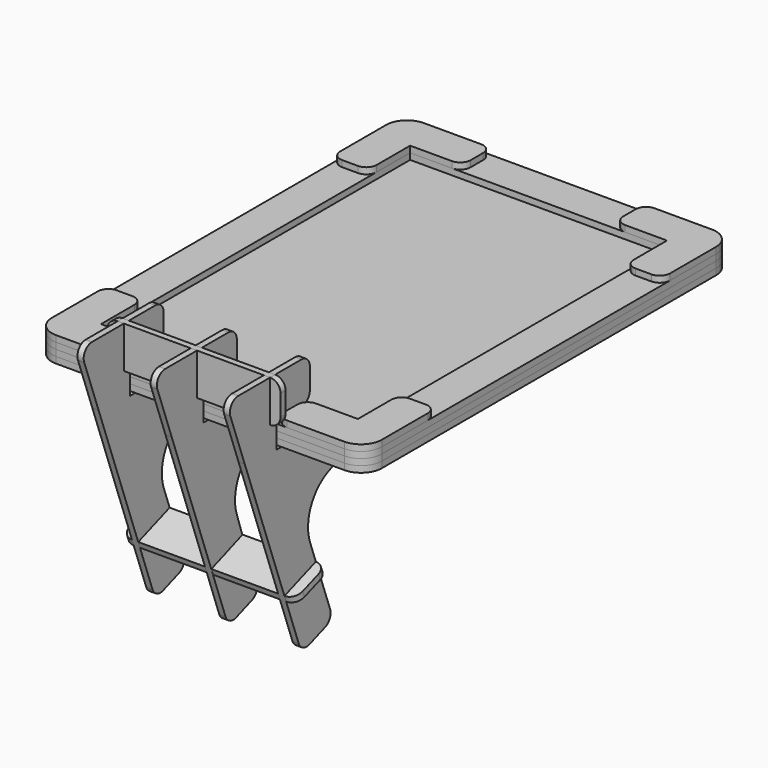
from build123d import *

# Parameters (mm, degrees)
F1_DEPTH  = 3
F3_R      = 6
F3_W      = 123
F3_H      = 185
F4_DEPTH  = 3
F5_R      = 6
F5_W      = 123
F5_H      = 185
F6_DEPTH  = 3
F9_DEPTH  = 1.5
F11_DEPTH = 1.5
F17_DEPTH = 3
F22_DEPTH = 3
F25_DEPTH = 3
F27_DEPTH = 3


# Not quite as in the source:
# - ends of sketch curves that miss each other by under 0.0002 mm in the source are joined


with BuildPart() as f1:
    # F0 (on Top) → F1 (new body)
    with BuildSketch(Plane.XY):
        with BuildLine():
            Line((-69, -110), (69, -110))
            ThreePointArc((69, -110), (76.0710678119, -107.0710678119), (79, -100))
            Line((79, -100), (79, 100))
            ThreePointArc((79, 100), (76.0710678119, 107.0710678119), (69, 110))
            Line((69, 110), (-69, 110))
            ThreePointArc((-69, 110), (-76.0710678119, 107.0710678119), (-79, 100))
            Line((-79, 100), (-79, -100))
            ThreePointArc((-79, -100), (-76.0710678119, -107.0710678119), (-69, -110))
        make_face()
    extrude(amount=F1_DEPTH)


with BuildPart() as f4:
    # F3 (on offset) → F4 (new body)
    with BuildSketch(Plane.XY.offset(3)):
        with BuildLine():
            Line((-69, -110), (69, -110))
            ThreePointArc((69, -110), (76.0710678119, -107.0710678119), (79, -100))
            Line((79, -100), (79, 100))
            ThreePointArc((79, 100), (76.0710678119, 107.0710678119), (69, 110))
            Line((69, 110), (-69, 110))
            ThreePointArc((-69, 110), (-76.0710678119, 107.0710678119), (-79, 100))
            Line((-79, 100), (-79, -100))
            ThreePointArc((-79, -100), (-76.0710678119, -107.0710678119), (-69, -110))
        make_face()
        with Locations((-68.7855339059, -99.7855339059)):
            Circle(F3_R, mode=Mode.SUBTRACT)
        with Locations((68.7855339059, -99.7855339059)):
            Circle(F3_R, mode=Mode.SUBTRACT)
        with Locations((-68.7855339059, 99.7855339059)):
            Circle(F3_R, mode=Mode.SUBTRACT)
        Rectangle(F3_W, F3_H, mode=Mode.SUBTRACT)
        with Locations((68.7855339059, 99.7855339059)):
            Circle(F3_R, mode=Mode.SUBTRACT)
    extrude(amount=F4_DEPTH)


with BuildPart() as f6:
    # F5 (on face) → F6 (new body)
    with BuildSketch(Plane(origin=(0, 0, 0), x_dir=(1, 0, 0), z_dir=(0, 0, -1))):
        with BuildLine():
            Line((-69, -110), (69, -110))
            ThreePointArc((69, -110), (76.0710678119, -107.0710678119), (79, -100))
            Line((79, -100), (79, 100))
            ThreePointArc((79, 100), (76.0710678119, 107.0710678119), (69, 110))
            Line((69, 110), (-69, 110))
            ThreePointArc((-69, 110), (-76.0710678119, 107.0710678119), (-79, 100))
            Line((-79, 100), (-79, -100))
            ThreePointArc((-79, -100), (-76.0710678119, -107.0710678119), (-69, -110))
        make_face()
        with Locations((-68.7855339059, -99.7855339059)):
            Circle(F5_R, mode=Mode.SUBTRACT)
        with Locations((68.7855339059, -99.7855339059)):
            Circle(F5_R, mode=Mode.SUBTRACT)
        with Locations((-68.7855339059, 99.7855339059)):
            Circle(F5_R, mode=Mode.SUBTRACT)
        Rectangle(F5_W, F5_H, mode=Mode.SUBTRACT)
        with Locations((68.7855339059, 99.7855339059)):
            Circle(F5_R, mode=Mode.SUBTRACT)
    extrude(amount=F6_DEPTH)


with BuildPart() as f9:
    # F8 (on offset) → F9 (new body, symmetric)
    with BuildSketch(Plane.YZ.offset(35)):
        with BuildLine():
            Line((-110, -5), (-110, 7))
            Line((-110, 7), (-95, 7))
            ThreePointArc((-95, 7), (-91.4644660941, 8.4644660941), (-90, 12))
            Line((-90, 12), (-90, 22))
            ThreePointArc((-90, 22), (-91.4644660941, 25.5355339059), (-95, 27))
            Line((-95, 27), (-111, 27))
            Line((-111, 27), (-111, 17))
            Line((-111, 17), (-113.8, 17))
            Line((-113.8, 17), (-113.8, 27))
            Line((-113.8, 27), (-132.8592599663, 27))
            ThreePointArc((-132.8592599663, 27), (-136.9550201877, 24.8678821818), (-137.5577230702, 20.2898992834))
            Line((-137.5577230702, 20.2898992834), (-128.9215966854, -3.4376629506))
            Line((-128.9215966854, -3.4376629506), (-96.6636040684, -92.0657692625))
            ThreePointArc((-96.6636040684, -92.0657692625), (-94.0782322732, -94.8872074811), (-90.2550402479, -95.0541316498))
            Line((-90.2550402479, -95.0541316498), (-80.85811404, -91.6339302166))
            ThreePointArc((-80.85811404, -91.6339302166), (-78.0366758215, -89.0485584213), (-77.8697516527, -85.225366396))
            Line((-77.8697516527, -85.225366396), (-85.4625988345, -64.3641902146))
            Line((-85.4625988345, -64.3641902146), (-94.8595250424, -67.7843916478))
            Line((-94.8595250424, -67.7843916478), (-95.8171814437, -65.1532523096))
            Line((-95.8171814437, -65.1532523096), (-86.4202552359, -61.7330508764))
            Line((-86.4202552359, -61.7330508764), (-89.8404566691, -52.3361246685))
            ThreePointArc((-89.8404566691, -52.3361246685), (-87.3851192861, -33.685985643), (-70.6994961108, -25))
            Line((-70.6994961108, -25), (-57.8, -24.9999998882))
            Line((-57.8, -24.9999998882), (-57.8, -14.9999998882))
            Line((-57.8, -14.9999998882), (-55, -14.9999998882))
            Line((-55, -14.9999998882), (-55, -24.9999998882))
            Line((-55, -24.9999998882), (-30, -24.9999998882))
            ThreePointArc((-30, -24.9999998882), (-26.4644660941, -23.5355337942), (-25, -19.9999998882))
            Line((-25, -19.9999998882), (-25, -6.9999998882))
            ThreePointArc((-25, -6.9999998882), (-26.4644660941, -3.4644659823), (-30, -1.9999998882))
            Line((-30, -1.9999998882), (-43.5, -1.9999998882))
            ThreePointArc((-43.5, -1.9999998882), (-44.5606601718, -2.4393397165), (-45, -3.4999998882))
            ThreePointArc((-45, -3.4999998882), (-45.4393398282, -4.56066006), (-46.5, -4.9999998882))
            Line((-46.5, -4.9999998882), (-110, -5))
        make_face()
    extrude(amount=F9_DEPTH, both=True)


with BuildPart() as f11:
    # F10 (on Right) → F11 (new body, symmetric)
    with BuildSketch(Plane.YZ):
        with BuildLine():
            Line((-110.7523969784, -8.8638670102), (-110.7523969784, 3.1361329898))
            Line((-110.7523969784, 3.1361329898), (-95.7523969784, 3.1361329898))
            ThreePointArc((-95.7523969784, 3.1361329898), (-92.2168630724, 4.6005990838), (-90.7523969784, 8.1361329898))
            Line((-90.7523969784, 8.1361329898), (-90.7523969784, 18.1361329898))
            ThreePointArc((-90.7523969784, 18.1361329898), (-92.2168630724, 21.6716668957), (-95.7523969784, 23.1361329898))
            Line((-95.7523969784, 23.1361329898), (-111.7523969784, 23.1361329898))
            Line((-111.7523969784, 23.1361329898), (-111.7523969784, 13.1361329898))
            Line((-111.7523969784, 13.1361329898), (-114.5523969784, 13.1361329898))
            Line((-114.5523969784, 13.1361329898), (-114.5523969784, 23.1361329898))
            Line((-114.5523969784, 23.1361329898), (-133.6116569447, 23.1361329898))
            ThreePointArc((-133.6116569447, 23.1361329898), (-137.7074171661, 21.0040151715), (-138.3101200486, 16.4260322731))
            Line((-138.3101200486, 16.4260322731), (-129.6739936637, -7.3015299608))
            Line((-129.6739936637, -7.3015299608), (-97.5212095615, -95.9682632155))
            ThreePointArc((-97.5212095615, -95.9682632155), (-94.9200677452, -98.7751693757), (-91.096000348, -98.9206667385))
            Line((-91.096000348, -98.9206667385), (-81.7183876115, -95.4478610478))
            ThreePointArc((-81.7183876115, -95.4478610478), (-78.9114814514, -92.8467192315), (-78.7659840886, -89.0226518343))
            Line((-78.7659840886, -89.0226518343), (-86.4756127218, -68.2043515593))
            Line((-86.4756127218, -68.2043515593), (-95.8532254583, -71.6771572499))
            Line((-95.8532254583, -71.6771572499), (-96.8256110516, -69.0514256837))
            Line((-96.8256110516, -69.0514256837), (-87.4479983152, -65.5786199931))
            Line((-87.4479983152, -65.5786199931), (-90.5928536475, -56.1999916787))
            ThreePointArc((-90.5928536475, -56.1999916787), (-88.1375162644, -37.5498526532), (-71.4518930892, -28.8638670102))
            Line((-71.4518930892, -28.8638670102), (-58.5523969784, -28.8638670102))
            Line((-58.5523969784, -28.8638670102), (-58.5523969784, -18.8638670102))
            Line((-58.5523969784, -18.8638670102), (-55.7523969784, -18.8638670102))
            Line((-55.7523969784, -18.8638670102), (-55.7523969784, -28.8638670102))
            Line((-55.7523969784, -28.8638670102), (-30.7523969784, -28.8638670102))
            ThreePointArc((-30.7523969784, -28.8638670102), (-27.2168630724, -27.3994009162), (-25.7523969784, -23.8638670102))
            Line((-25.7523969784, -23.8638670102), (-25.7523969784, -10.8638670102))
            ThreePointArc((-25.7523969784, -10.8638670102), (-27.2168630724, -7.3283331043), (-30.7523969784, -5.8638670102))
            Line((-30.7523969784, -5.8638670102), (-44.2523969784, -5.8638670102))
            ThreePointArc((-44.2523969784, -5.8638670102), (-45.3130571501, -6.3032068385), (-45.7523969784, -7.3638670102))
            ThreePointArc((-45.7523969784, -7.3638670102), (-46.1917368066, -8.424527182), (-47.2523969784, -8.8638670102))
            Line((-47.2523969784, -8.8638670102), (-110.7523969784, -8.8638670102))
        make_face()
    extrude(amount=F11_DEPTH, both=True)


with BuildPart() as f11_1:
    # F12: moved
    add(f11.part.moved(Location((0, 0, 4))))


with BuildPart() as f13_1:
    # F13: instance of F9
    add(f9.part.mirror(Plane.YZ))


with BuildPart() as f11_2:
    # F16: moved
    add(f11_1.part.moved(Location((0, 0, 0.136))))


with BuildPart() as f17:
    # F15 (on offset) → F17 (new body)
    with BuildSketch(Plane(origin=(0, -113.8, 0), x_dir=(-1, 0, 0), z_dir=(0, 1, 0))):
        with BuildLine():
            Line((-1.5, 7), (-1.5, 17))
            Line((-1.5, 17), (1.5, 17))
            Line((1.5, 17), (1.5, 7))
            Line((1.5, 7), (33.5, 7.0000009239))
            Line((33.5, 7.0000009239), (33.5, 17.0000009239))
            Line((33.5, 17.0000009239), (36.5, 17.0000009239))
            Line((36.5, 17.0000009239), (36.5, 7.0000009239))
            ThreePointArc((36.5, 7.0000009239), (40.0355339059, 8.4644670179), (41.5, 12.0000009239))
            Line((41.5, 12.0000009239), (41.5, 22.0000009239))
            ThreePointArc((41.5, 22.0000009239), (40.0355339059, 25.5355348298), (36.5, 27.0000009239))
            Line((36.5, 27.0000009239), (-36.5, 27.0000009239))
            ThreePointArc((-36.5, 27.0000009239), (-40.0355339059, 25.5355348298), (-41.5, 22.0000009239))
            Line((-41.5, 22.0000009239), (-41.5, 12.0000009239))
            ThreePointArc((-41.5, 12.0000009239), (-40.0355339059, 8.4644670179), (-36.5, 7.0000009239))
            Line((-36.5, 7.0000009239), (-36.5, 17.0000009239))
            Line((-36.5, 17.0000009239), (-33.5, 17.0000009239))
            Line((-33.5, 17.0000009239), (-33.5, 7.0000009239))
            Line((-33.5, 7.0000009239), (-1.5, 7))
        make_face()
    extrude(amount=F17_DEPTH)


with BuildPart() as f11_3:
    # F18: moved
    add(f11_2.part.moved(Location((0, 0.2, -0.272))))


with BuildPart() as f11_4:
    # F19: moved
    add(f11_3.part.moved(Location((0, 0.6, 0))))


with BuildPart() as f22:
    # F21 (on offset) → F22 (new body)
    with BuildSketch(Plane(origin=(0, 9.731370636, -26.7367210827), x_dir=(1, 0, 0), z_dir=(0, 0.3420201433, -0.9396926208))):
        with BuildLine():
            Line((1.5, 122.3224239641), (1.5, 112.3224239641))
            Line((1.5, 112.3224239641), (-1.5, 112.3224239641))
            Line((-1.5, 112.3224239641), (-1.5, 122.3224239641))
            Line((-1.5, 122.3224239641), (-33.5, 122.3224230402))
            Line((-33.5, 122.3224230402), (-33.5, 112.3224230402))
            Line((-33.5, 112.3224230402), (-36.5, 112.3224230402))
            Line((-36.5, 112.3224230402), (-36.5, 122.3224230402))
            ThreePointArc((-36.5, 122.3224230402), (-40.0355339059, 120.8579569462), (-41.5, 117.3224230402))
            Line((-41.5, 117.3224230402), (-41.5, 107.3224230402))
            ThreePointArc((-41.5, 107.3224230402), (-40.0355339059, 103.7868891343), (-36.5, 102.3224230402))
            Line((-36.5, 102.3224230402), (36.5, 102.3224230402))
            ThreePointArc((36.5, 102.3224230402), (40.0355339059, 103.7868891343), (41.5, 107.3224230402))
            Line((41.5, 107.3224230402), (41.5, 117.3224230402))
            ThreePointArc((41.5, 117.3224230402), (40.0355339059, 120.8579569462), (36.5, 122.3224230402))
            Line((36.5, 122.3224230402), (36.5, 112.3224230402))
            Line((36.5, 112.3224230402), (33.5, 112.3224230402))
            Line((33.5, 112.3224230402), (33.5, 122.3224230402))
            Line((33.5, 122.3224230402), (1.5, 122.3224239641))
        make_face()
    extrude(amount=F22_DEPTH)


with BuildPart() as f25:
    # F24 (on offset) → F25 (new body)
    with BuildSketch(Plane(origin=(0, -57.8, 0), x_dir=(-1, 0, 0), z_dir=(0, 1, 0))):
        with BuildLine():
            ThreePointArc((-36.4999994636, -5.0000009239), (-40.0355333695, -6.4644670179), (-41.4999994636, -10.0000009239))
            Line((-41.4999994636, -10.0000009239), (-41.4999994636, -20.0000009239))
            ThreePointArc((-41.4999994636, -20.0000009239), (-40.0355333695, -23.5355348298), (-36.4999994636, -25.0000009239))
            Line((-36.4999994636, -25.0000009239), (-33.4999994636, -25.0000019595))
            Line((-33.4999994636, -25.0000019595), (-1.4999994636, -25.0000009239))
            Line((-1.4999994636, -25.0000009239), (1.5000005364, -25.0000019595))
            Line((1.5000005364, -25.0000019595), (33.5000005364, -25.0000009239))
            Line((33.5000005364, -25.0000009239), (36.5000005364, -25.0000019595))
            ThreePointArc((36.5000005364, -25.0000019595), (40.0355344424, -23.5355348298), (41.5000005364, -20.0000009239))
            Line((41.5000005364, -20.0000009239), (41.5000005364, -10.0000009239))
            ThreePointArc((41.5000005364, -10.0000009239), (40.0355344424, -6.4644670179), (36.5000005364, -5.0000009239))
            Line((36.5000005364, -5.0000009239), (36.5000005364, -15.0000009239))
            Line((36.5000005364, -15.0000009239), (33.5000005364, -15.0000009239))
            Line((33.5000005364, -15.0000009239), (33.5000005364, -5.0000009239))
            Line((33.5000005364, -5.0000009239), (1.5000005364, -5.0000009239))
            Line((1.5000005364, -5.0000009239), (1.5000005364, -15.0000009239))
            Line((1.5000005364, -15.0000009239), (-1.4999994636, -15.0000009239))
            Line((-1.4999994636, -15.0000009239), (-1.4999994636, -5.0000009239))
            Line((-1.4999994636, -5.0000009239), (-33.4999994636, -5.0000009239))
            Line((-33.4999994636, -5.0000009239), (-33.4999994636, -15.0000009239))
            Line((-33.4999994636, -15.0000009239), (-36.4999994636, -15.0000019595))
            Line((-36.4999994636, -15.0000019595), (-36.4999994636, -5.0000009239))
        make_face()
    extrude(amount=F25_DEPTH)


with BuildPart() as f27:
    # F26 (on face) → F27 (new body)
    with BuildSketch(Plane.XY.offset(6)):
        with BuildLine():
            Line((-79, -72.5), (-79, -100))
            ThreePointArc((-79, -100), (-76.0710678119, -107.0710678119), (-69, -110))
            Line((-69, -110), (-41.5, -110))
            ThreePointArc((-41.5, -110), (-37.9644660941, -108.5355339059), (-36.5, -105))
            Line((-36.5, -105), (-36.5, -97.5))
            ThreePointArc((-36.5, -97.5), (-37.9644660941, -93.9644660941), (-41.5, -92.5))
            Line((-41.5, -92.5), (-61.5, -92.5))
            Line((-61.5, -92.5), (-61.5, -72.5))
            ThreePointArc((-61.5, -72.5), (-62.9644660941, -68.9644660941), (-66.5, -67.5))
            Line((-66.5, -67.5), (-74, -67.5))
            ThreePointArc((-74, -67.5), (-77.5355339059, -68.9644660941), (-79, -72.5))
        make_face()
    extrude(amount=F27_DEPTH)


with BuildPart() as f27b:
    # F26 (on face) → F27, piece 2 (new body)
    with BuildSketch(Plane.XY.offset(6)):
        with BuildLine():
            Line((61.5, -92.5), (41.5, -92.5))
            ThreePointArc((41.5, -92.5), (37.9644660941, -93.9644660941), (36.5, -97.5))
            Line((36.5, -97.5), (36.5, -105))
            ThreePointArc((36.5, -105), (37.9644660941, -108.5355339059), (41.5, -110))
            Line((41.5, -110), (69, -110))
            ThreePointArc((69, -110), (76.0710678119, -107.0710678119), (79, -100))
            Line((79, -100), (79, -72.5))
            ThreePointArc((79, -72.5), (77.5355339059, -68.9644660941), (74, -67.5))
            Line((74, -67.5), (66.5, -67.5))
            ThreePointArc((66.5, -67.5), (62.9644660941, -68.9644660941), (61.5, -72.5))
            Line((61.5, -72.5), (61.5, -92.5))
        make_face()
    extrude(amount=F27_DEPTH)


with BuildPart() as f27c:
    # F26 (on face) → F27, piece 3 (new body)
    with BuildSketch(Plane.XY.offset(6)):
        with BuildLine():
            Line((-36.5, 97.5), (-36.5, 105))
            ThreePointArc((-36.5, 105), (-37.9644660941, 108.5355339059), (-41.5, 110))
            Line((-41.5, 110), (-69, 110))
            ThreePointArc((-69, 110), (-76.0710678119, 107.0710678119), (-79, 100))
            Line((-79, 100), (-79, 72.5))
            ThreePointArc((-79, 72.5), (-77.5355339059, 68.9644660941), (-74, 67.5))
            Line((-74, 67.5), (-66.5, 67.5))
            ThreePointArc((-66.5, 67.5), (-62.9644660941, 68.9644660941), (-61.5, 72.5))
            Line((-61.5, 72.5), (-61.5, 92.5))
            Line((-61.5, 92.5), (-41.5, 92.5))
            ThreePointArc((-41.5, 92.5), (-37.9644660941, 93.9644660941), (-36.5, 97.5))
        make_face()
    extrude(amount=F27_DEPTH)


with BuildPart() as f27d:
    # F26 (on face) → F27, piece 4 (new body)
    with BuildSketch(Plane.XY.offset(6)):
        with BuildLine():
            ThreePointArc((36.5, 97.5), (37.9644660941, 93.9644660941), (41.5, 92.5))
            Line((41.5, 92.5), (61.5, 92.5))
            Line((61.5, 92.5), (61.5, 72.5))
            ThreePointArc((61.5, 72.5), (62.9644660941, 68.9644660941), (66.5, 67.5))
            Line((66.5, 67.5), (74, 67.5))
            ThreePointArc((74, 67.5), (77.5355339059, 68.9644660941), (79, 72.5))
            Line((79, 72.5), (79, 100))
            ThreePointArc((79, 100), (76.0710678119, 107.0710678119), (69, 110))
            Line((69, 110), (41.5, 110))
            ThreePointArc((41.5, 110), (37.9644660941, 108.5355339059), (36.5, 105))
            Line((36.5, 105), (36.5, 97.5))
        make_face()
    extrude(amount=F27_DEPTH)


solid = Compound([f1.part, f4.part, f6.part, f9.part, f13_1.part, f17.part, f11_4.part, f22.part, f25.part, f27.part, f27b.part, f27c.part, f27d.part])
